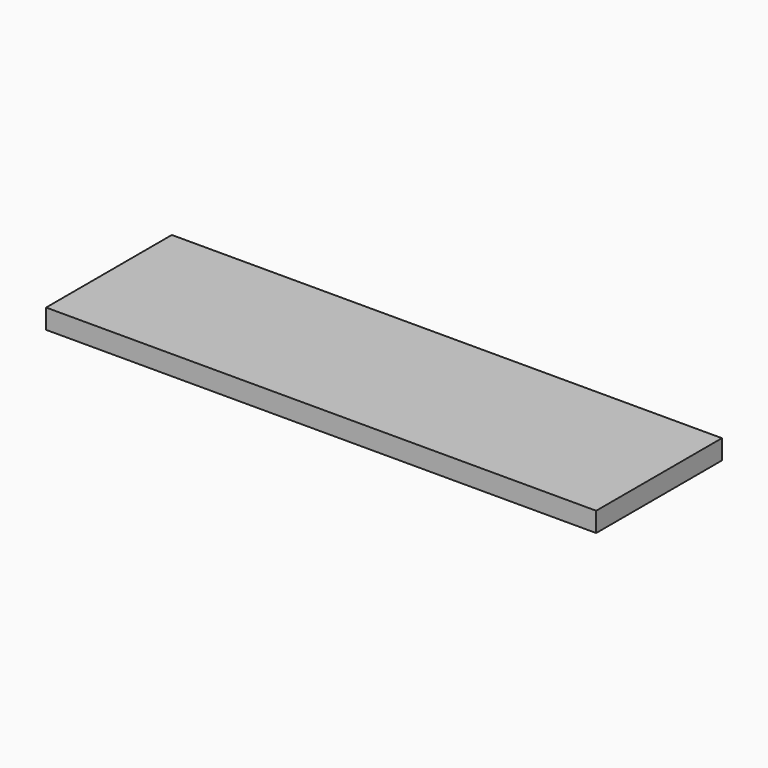
from build123d import *

# Parameters (mm, degrees)
F1_W     = 177.8
F1_H     = 50.8
F2_DEPTH = 6.35


# Not quite as in the source:
# - a variable given as a bare number and used for a length is read in inches; the dataset says mm whatever the document's units were


with BuildPart() as f2:
    # F1 (on Top) → F2 (new body)
    with BuildSketch(Plane.XY):
        with Locations((88.9, 25.4)):
            Rectangle(F1_W, F1_H)
    extrude(amount=F2_DEPTH)


solid = f2.part
